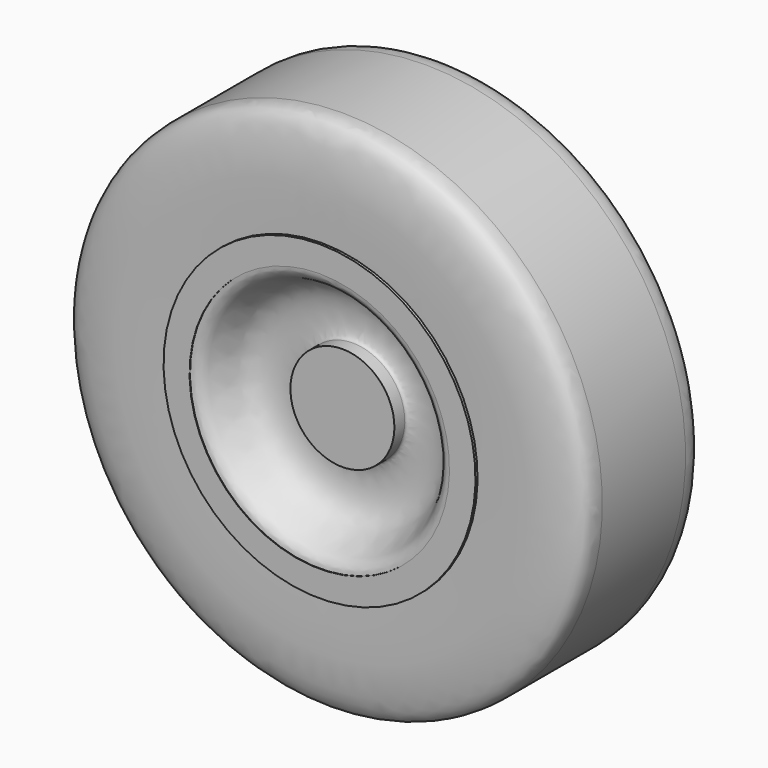
from build123d import *

# Parameters (mm, degrees)
F4_SCALE = 1.3


# Not quite as in the source:
# - ends of sketch curves that miss each other by under 0.0002 mm in the source are joined
# - a feature of the source that left no trace in its solid (it failed there, or was rolled back) is left out


with BuildPart() as f1:
    # F0 (on Right) → F1 (revolve)
    with BuildSketch(Plane.YZ):
        with BuildLine():
            Line((-10, 10), (-10, 0))
            Line((-10, 0), (10, 0))
            Line((10, 0), (10, 10))
            Line((10, 10), (7.5, 10))
            add(Edge.make_bspline(
                [(7.5, 10), (6.3198292539, 10.0170777093), (6.0755360942, 16.2900794914), (8.71740503, 20.4397404153), (14.1975799439, 22.3834382863), (15.4026740679, 23.9286791718), (15.4000005056, 25)],
                knots=[0, 0, 0, 0, 0.2720899799, 0.5413764913, 0.8105016424, 1, 1, 1, 1], degree=3))
            Line((15.4000005056, 25), (15.5000005056, 25))
            Line((15.5000005056, 25), (15.5000005056, 30))
            Line((15.5000005056, 30), (15.0000005056, 30))
            add(Edge.make_bspline(
                [(15.0000005056, 30), (15.0842336639, 34.1735254493), (15.4036855603, 41.6818231934), (14.026949329, 49.0386767347), (12.0611475076, 50.0140784293), (10.0000005056, 50)],
                knots=[0, 0, 0, 0, 0.4362070764, 0.7559396549, 1, 1, 1, 1], degree=3))
            Line((10.0000005056, 50), (5.056e-07, 50))
            Line((5.056e-07, 50), (-10.0000005056, 50))
            add(Edge.make_bspline(
                [(-15.0000005056, 30), (-15.0842336639, 34.1735254493), (-15.4036855603, 41.6818231934), (-14.026949329, 49.0386767347), (-12.0611475076, 50.0140784293), (-10.0000005056, 50)],
                knots=[0, 0, 0, 0, 0.4362070764, 0.7559396549, 1, 1, 1, 1], degree=3))
            Line((-15.0000005056, 30), (-15.5000005056, 30))
            Line((-15.5000005056, 30), (-15.5000005056, 25))
            Line((-15.5000005056, 25), (-15.4000005056, 25))
            add(Edge.make_bspline(
                [(-7.5, 10), (-6.3198292539, 10.0170777093), (-6.0755360942, 16.2900794914), (-8.71740503, 20.4397404153), (-14.1975799439, 22.3834382863), (-15.4026740679, 23.9286791718), (-15.4000005056, 25)],
                knots=[0, 0, 0, 0, 0.2720899799, 0.5413764913, 0.8105016424, 1, 1, 1, 1], degree=3))
            Line((-7.5, 10), (-10, 10))
        make_face()
    revolve(axis=Axis((0, 0, 0), (0, 1, 0)))


with BuildPart() as f1_1:
    # F4: moved
    add(f1.part.scale(F4_SCALE))


solid = f1_1.part
